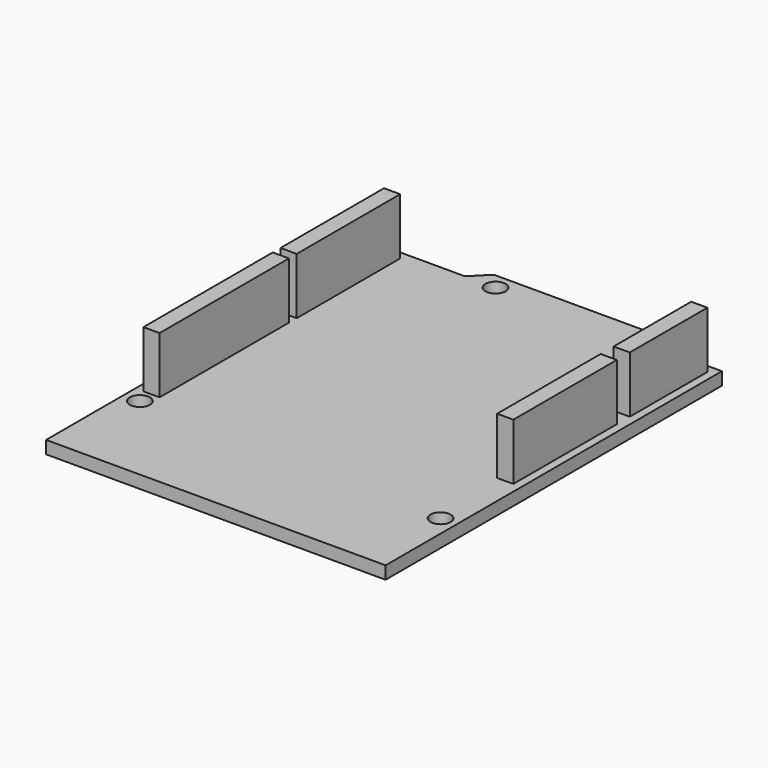
from build123d import *

# Parameters (mm, degrees)
F0_W     = 53.34
F0_H     = 68.58
F1_DEPTH = 2
F3_DEPTH = 2
F6_D     = 3.175
F7_W     = 2.54
F7_H     = 20.32
F7_H_2   = 25.4
F7_H_3   = 15.24
F8_DEPTH = 8.89


# Not quite as in the source:
# - a feature names something its author has since deleted; it is built from what else it names


with BuildPart() as f1:
    # F0 (on Top) → F1 (new body)
    with BuildSketch(Plane.XY):
        Rectangle(F0_W, F0_H)
    extrude(amount=-F1_DEPTH)

    # F2 (on face) → F3 (cut, through all)
    with BuildSketch(Plane.XY):
        Polygon((-25.146, 31.75), (-13.716, 31.75), (-11.176, 34.29), (-26.67, 34.29), (-26.67, 30.226), align=None)
        Polygon((26.67, 34.29), (21.59, 34.29), (24.13, 31.75), (26.67, 31.75), align=None)
    extrude(amount=-F3_DEPTH, mode=Mode.SUBTRACT)

    # F6 (through all)
    with Locations(Plane.XY):
        with Locations((-24.13, -19.05), (24.13, -20.32), (19.05, 31.75), (-8.89, 31.75)):
            Hole(F6_D / 2)

    # F7 (on face) → F8 (join)
    with BuildSketch(Plane.XY):
        with Locations((-24.13, 20.32)):
            Rectangle(F7_W, F7_H)
        with Locations((-24.13, -4.064)):
            Rectangle(F7_W, F7_H_2)
        with Locations((24.13, 22.86)):
            Rectangle(F7_W, F7_H_3)
        with Locations((24.13, 2.54)):
            Rectangle(F7_W, F7_H)
    extrude(amount=F8_DEPTH)


solid = f1.part
